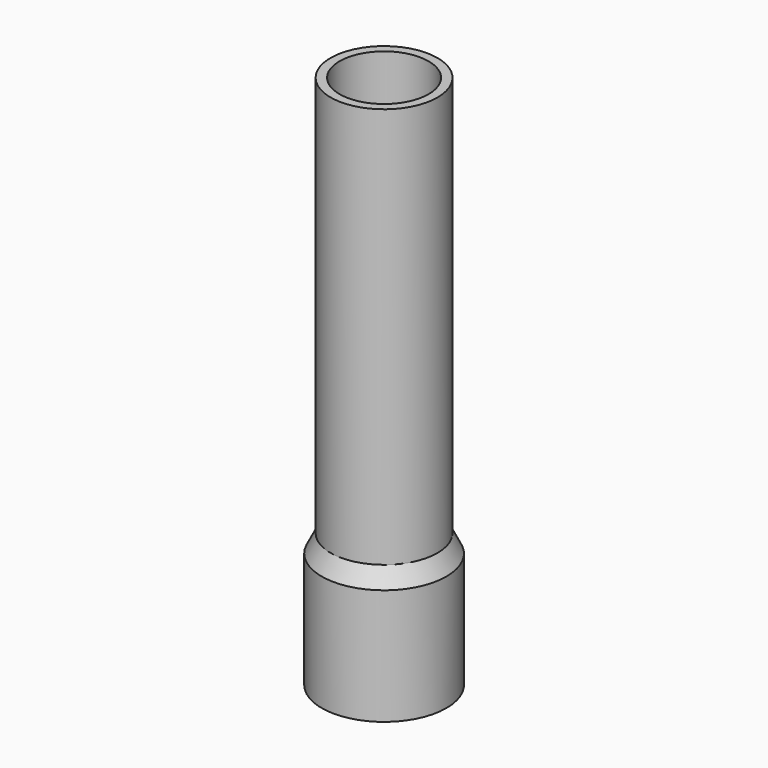
from build123d import *

# Parameters (mm, degrees)
F0_R     = 17.78
F1_DEPTH = 38.1
F2_R     = 15.24
F3_DEPTH = 114.3
F4_R     = 15.24
F5_DEPTH = 31.75
F6_R     = 12.7
F7_DEPTH = 127
F8_SIZE2 = 5.07999
F8_SIZE  = 2.53999


# Not quite as in the source:
# - a fillet or chamfer is up to 0.001 mm smaller than in the source, because OpenCascade refuses the exact size


with BuildPart() as f1:
    # F0 (on Top) → F1 (new body)
    with BuildSketch(Plane.XY):
        Circle(F0_R)
    extrude(amount=F1_DEPTH)

    # F2 (on face) → F3 (join)
    with BuildSketch(Plane.XY.offset(38.1)):
        Circle(F2_R)
    extrude(amount=F3_DEPTH)

    # F4 (on face) → F5 (cut)
    with BuildSketch(Plane(origin=(0, 0, 0), x_dir=(1, 0, 0), z_dir=(0, 0, -1))):
        Circle(F4_R)
    extrude(amount=-F5_DEPTH, mode=Mode.SUBTRACT)

    # F6 (on face) → F7 (cut)
    with BuildSketch(Plane.XY.offset(152.4)):
        Circle(F6_R)
    extrude(amount=-F7_DEPTH, mode=Mode.SUBTRACT)

    # F8 (size 2.54 and 5.08 in the source; OpenCascade refuses exactly that, so slightly less here)
    f8_edges = [f1.edges().sort_by_distance(p)[0] for p in [
        (-17.78, 0, 38.1),
    ]]
    f8_side = f1.faces().sort_by_distance((-17.277106, 0, 38.1))[0]
    chamfer(f8_edges, length=F8_SIZE, length2=F8_SIZE2, reference=f8_side)


solid = f1.part
